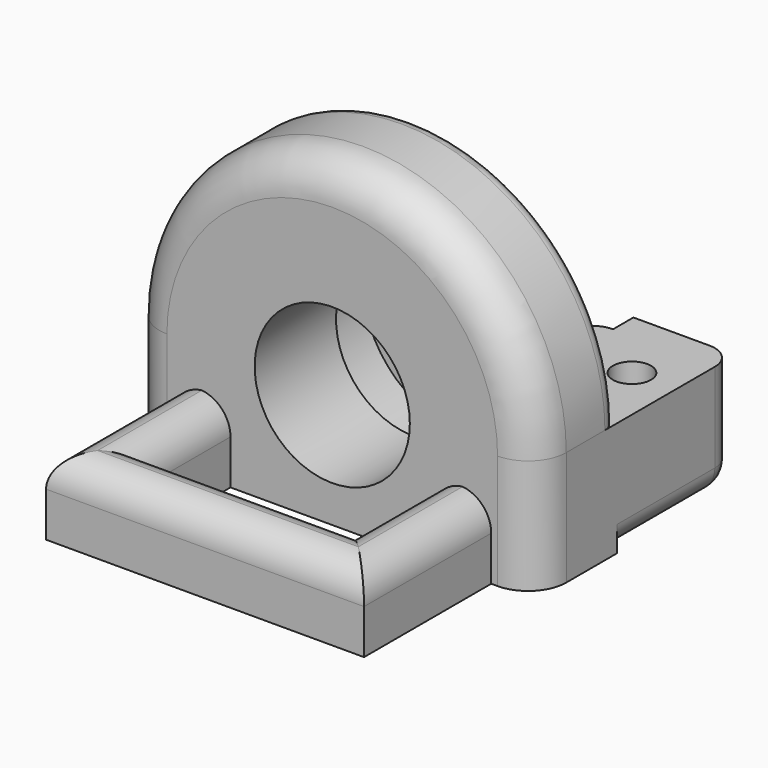
from build123d import *

# Parameters (mm, degrees)
F0_W          = 32
F0_H          = 11.6
F0_R          = 1.5
F1_DEPTH      = 9
F2_R          = 8
F1_FACE1_W    = 32
F1_FACE1_H    = 9
F3_DEPTH      = 5
F4_R          = 8
F5_DEPTH      = 2
F6_R          = 6
F7_DEPTH      = 25
F8_T1_DEPTH   = 28
F8_T3_DEPTH   = 12
F8_T5_DEPTH   = 14.6
F8_S9_W       = 2
F8_S9_H       = 2
F8_T10_DEPTH  = 2
F8_S15_W      = 2
F8_S15_H      = 2
F8_T16_DEPTH  = 2
F8_T20_ANGLE  = 275.6465366004
F10_DEPTH     = 8
F12_DEPTH     = 6
F13_T1_DEPTH  = 8
F13_T3_DEPTH  = 18.75
F13_T5_DEPTH  = 16
F13_T7_DEPTH  = 37.5
F13_T13_DEPTH = 14.25
F13_T17_DEPTH = 22.25
F13_T24_DEPTH = 14.25
F13_T28_DEPTH = 22.25
F14_R         = 3
F15_R         = 1.2
F16_R         = 6.1
F17_DEPTH     = 19.6010001
F18_T3_ANGLE  = 90
F18_T6_DEPTH  = 10
F18_T9_DEPTH  = 0.5


# Not quite as in the source:
# - a fillet or chamfer that OpenCascade refuses, or shapes differently, is made with other operations: its cross-section is extruded or revolved along the edge and cut away or added


with BuildPart() as f1:
    # F0 (on Top) → F1 (new body)
    with BuildSketch(Plane.XY):
        Rectangle(F0_W, F0_H)
        with Locations((-12.524, 0)):
            Circle(F0_R, mode=Mode.SUBTRACT)
        with Locations((12.524, 0)):
            Circle(F0_R, mode=Mode.SUBTRACT)
    extrude(amount=F1_DEPTH)

    # F2 (on face) + F1_face1 (on face) → F3 (cut)
    with BuildSketch(Plane.XZ.offset(5.8)):
        with Locations((0, 9)):
            Circle(F2_R)
    with BuildSketch(Plane(origin=(0, 5.8, 4.5), x_dir=(-1, 0, 0), z_dir=(0, 1, 0))):
        Rectangle(F1_FACE1_W, F1_FACE1_H)
    extrude(amount=-F3_DEPTH, dir=(0, -1, 0), mode=Mode.SUBTRACT)

    # F4 (on face) → F5 (cut)
    with BuildSketch(Plane(origin=(0, 5.8, 0), x_dir=(-1, 0, 0), z_dir=(0, 1, 0))):
        with Locations((0, 9)):
            Circle(F4_R)
    extrude(amount=-F5_DEPTH, mode=Mode.SUBTRACT)

    # F6 (on face) → F7 (cut)
    with BuildSketch(Plane(origin=(0, 3.8, 0), x_dir=(-1, 0, 0), z_dir=(0, 1, 0))):
        with Locations((0, 9)):
            Circle(F6_R)
    extrude(amount=-F7_DEPTH, mode=Mode.SUBTRACT)

    # F8: fillet of radius 2 on 6 edges, made by hand

    # F8_s2 → F8_t1 (cut)
    with BuildSketch(Plane.YZ.offset(-14)):
        with BuildLine():
            ThreePointArc((5.8, 2), (5.2142135624, 0.5857864376), (3.8, 0))
            Line((3.8, 0), (5.8, 0))
            Line((5.8, 0), (5.8, 2))
        make_face()
    extrude(amount=F8_T1_DEPTH, mode=Mode.SUBTRACT)

    # F8_s4 → F8_t3 (cut)
    with BuildSketch(Plane.XY.offset(2)):
        with BuildLine():
            ThreePointArc((-14, 5.8), (-15.4142135624, 5.2142135624), (-16, 3.8))
            Line((-16, 3.8), (-16, 5.8))
            Line((-16, 5.8), (-14, 5.8))
        make_face()
        with BuildLine():
            ThreePointArc((14, 5.8), (15.4142135624, 5.2142135624), (16, 3.8))
            Line((16, 3.8), (16, 5.8))
            Line((16, 5.8), (14, 5.8))
        make_face()
    extrude(amount=F8_T3_DEPTH, mode=Mode.SUBTRACT)

    # F8_s6 → F8_t5 (cut)
    with BuildSketch(Plane.XZ.offset(-3.8)):
        with BuildLine():
            ThreePointArc((-14, 0), (-15.4142135624, 0.5857864376), (-16, 2))
            Line((-16, 2), (-16, 0))
            Line((-16, 0), (-14, 0))
        make_face()
        with BuildLine():
            ThreePointArc((14, 0), (15.4142135624, 0.5857864376), (16, 2))
            Line((16, 2), (16, 0))
            Line((16, 0), (14, 0))
        make_face()
    extrude(amount=F8_T5_DEPTH, mode=Mode.SUBTRACT)


with BuildPart() as f8_tool8:
    # F8_s9 → F8_t10 (new body)
    with BuildSketch(Plane.XZ.offset(-3.8)):
        with Locations((15, 1)):
            Rectangle(F8_S9_W, F8_S9_H)
    extrude(amount=-F8_T10_DEPTH)

    # F8_s11 → F8_t12 (revolve, cut)
    with BuildSketch(Plane(origin=(14, 3.8, 2), x_dir=(-0.7071067812, 0, 0.7071067812), z_dir=(-0.7071067812, 0, -0.7071067812))):
        with BuildLine():
            ThreePointArc((0, -2), (2, 0), (0, 2))
            Line((0, 2), (0, -2))
        make_face()
    revolve(axis=Axis((14, 3.8, 2), (0, 1, 0)), mode=Mode.SUBTRACT)


with BuildPart() as f1_1:
    add(f1.part)

    # F8_t7: cut F8_tool8
    add(f8_tool8.part, mode=Mode.SUBTRACT)


with BuildPart() as f8_tool14:
    # F8_s15 → F8_t16 (new body)
    with BuildSketch(Plane.XZ.offset(-3.8)):
        with Locations((-15, 1)):
            Rectangle(F8_S15_W, F8_S15_H)
    extrude(amount=-F8_T16_DEPTH)

    # F8_s17 → F8_t18 (revolve, cut)
    with BuildSketch(Plane(origin=(-14, 3.8, 2), x_dir=(0.7071067812, 0, 0.7071067812), z_dir=(-0.7071067812, 0, 0.7071067812))):
        with BuildLine():
            ThreePointArc((0, -2), (2, 0), (0, 2))
            Line((0, 2), (0, -2))
        make_face()
    revolve(axis=Axis((-14, 3.8, 2), (0, 1, 0)), mode=Mode.SUBTRACT)


with BuildPart() as f1_2:
    add(f1_1.part)

    # F8_t13: cut F8_tool14
    add(f8_tool14.part, mode=Mode.SUBTRACT)

    # F8_s19 → F8_t20 (revolve, cut)
    with BuildSketch(Plane(origin=(-4.4781651596, 0, 4.057239564), x_dir=(0, 1, 0), z_dir=(-0.7410773266, 0, 0.6714196869))):
        with BuildLine():
            ThreePointArc((3.8, -14.6696959394), (3.2142135624, -13.255482377), (1.8, -12.6696959394))
            Line((1.8, -12.6696959394), (3.8, -12.6696959394))
            Line((3.8, -12.6696959394), (3.8, -14.6696959394))
        make_face()
    revolve(axis=Axis((0, 3.8, 9), (0, 1, 0)), revolution_arc=F8_T20_ANGLE, mode=Mode.SUBTRACT)

    # F9 (on face) → F10 (join)
    with BuildSketch(Plane.XZ.offset(5.8)):
        with BuildLine():
            Line((16, 0), (16, 9))
            ThreePointArc((16, 9), (0, 25), (-16, 9))
            Line((-16, 9), (-16, 0))
            Line((-16, 0), (-13.2287565553, 0))
            Line((-13.2287565553, 0), (0, 0))
            Line((0, 0), (13.2287565553, 0))
            Line((13.2287565553, 0), (16, 0))
        make_face()
    extrude(amount=F10_DEPTH)

    # F11 (on Top) → F12 (join)
    with BuildSketch(Plane.XY):
        Polygon((-8, -21.8), (-8, -13.8), (-12.5, -13.8), (-12.5, -26.3), (12.5, -26.3), (12.5, -13.8), (8, -13.8), (8, -21.8), align=None)
    extrude(amount=F12_DEPTH)

    # F13: fillet of radius 2.5 on 6 edges, made by hand

    # F13_s2 → F13_t1 (cut)
    with BuildSketch(Plane.XZ.offset(13.8)):
        with BuildLine():
            ThreePointArc((-10.5, 6), (-8.732233047, 5.267766953), (-8, 3.5))
            Line((-8, 3.5), (-8, 6))
            Line((-8, 6), (-10.5, 6))
        make_face()
        with BuildLine():
            ThreePointArc((10.5, 6), (8.732233047, 5.267766953), (8, 3.5))
            Line((8, 3.5), (8, 6))
            Line((8, 6), (10.5, 6))
        make_face()
    extrude(amount=F13_T1_DEPTH, mode=Mode.SUBTRACT)

    # F13_s4 → F13_t3 (cut)
    with BuildSketch(Plane.XZ.offset(13.8)):
        with BuildLine():
            ThreePointArc((-10, 6), (-11.767766953, 5.267766953), (-12.5, 3.5))
            Line((-12.5, 3.5), (-12.5, 6))
            Line((-12.5, 6), (-10, 6))
        make_face()
        with BuildLine():
            ThreePointArc((12.5, 3.5), (11.767766953, 5.267766953), (10, 6))
            Line((10, 6), (12.5, 6))
            Line((12.5, 6), (12.5, 3.5))
        make_face()
    extrude(amount=F13_T3_DEPTH, mode=Mode.SUBTRACT)

    # F13_s6 → F13_t5 (cut)
    with BuildSketch(Plane.YZ.offset(-8)):
        with BuildLine():
            ThreePointArc((-24.3, 6), (-22.532233047, 5.267766953), (-21.8, 3.5))
            Line((-21.8, 3.5), (-21.8, 6))
            Line((-21.8, 6), (-24.3, 6))
        make_face()
    extrude(amount=F13_T5_DEPTH, mode=Mode.SUBTRACT)

    # F13_s8 → F13_t7 (cut)
    with BuildSketch(Plane.YZ.offset(-18.75)):
        with BuildLine():
            ThreePointArc((-23.8, 6), (-25.567766953, 5.267766953), (-26.3, 3.5))
            Line((-26.3, 3.5), (-26.3, 6))
            Line((-26.3, 6), (-23.8, 6))
        make_face()
    extrude(amount=F13_T7_DEPTH, mode=Mode.SUBTRACT)


with BuildPart() as f13_tool11:
    # F13_s12 → F13_t13 (new body)
    with BuildSketch(Plane.XZ.offset(28.05)):
        with BuildLine():
            ThreePointArc((-10.5, 6), (-8.732233047, 5.267766953), (-8, 3.5))
            Line((-8, 3.5), (-8, 6))
            Line((-8, 6), (-10.5, 6))
        make_face()
    extrude(amount=-F13_T13_DEPTH)

    split(bisect_by=Plane.XZ.offset(21.8), keep=Keep.TOP)


with BuildPart() as f13_tool15:
    # F13_s16 → F13_t17 (new body)
    with BuildSketch(Plane.YZ.offset(8)):
        with BuildLine():
            ThreePointArc((-24.3, 6), (-22.532233047, 5.267766953), (-21.8, 3.5))
            Line((-21.8, 3.5), (-21.8, 6))
            Line((-21.8, 6), (-24.3, 6))
        make_face()
    extrude(amount=-F13_T17_DEPTH)

    split(bisect_by=Plane.YZ.offset(-8), keep=Keep.BOTTOM)


with BuildPart() as f13_tool11_1:
    add(f13_tool11.part)

    # F13_t19: intersect F13_tool15
    add(f13_tool15.part, mode=Mode.INTERSECT)


with BuildPart() as f1_3:
    add(f1_2.part)

    # F13_t9: cut F13_tool11
    add(f13_tool11_1.part, mode=Mode.SUBTRACT)


with BuildPart() as f13_tool22:
    # F13_s23 → F13_t24 (new body)
    with BuildSketch(Plane.XZ.offset(13.8)):
        with BuildLine():
            ThreePointArc((10.5, 6), (8.732233047, 5.267766953), (8, 3.5))
            Line((8, 3.5), (8, 6))
            Line((8, 6), (10.5, 6))
        make_face()
    extrude(amount=F13_T24_DEPTH)

    split(bisect_by=Plane.XZ.offset(21.8), keep=Keep.TOP)


with BuildPart() as f13_tool26:
    # F13_s27 → F13_t28 (new body)
    with BuildSketch(Plane.YZ.offset(14.25)):
        with BuildLine():
            ThreePointArc((-24.3, 6), (-22.532233047, 5.267766953), (-21.8, 3.5))
            Line((-21.8, 3.5), (-21.8, 6))
            Line((-21.8, 6), (-24.3, 6))
        make_face()
    extrude(amount=-F13_T28_DEPTH)

    split(bisect_by=Plane.YZ.offset(8), keep=Keep.TOP)


with BuildPart() as f13_tool22_1:
    add(f13_tool22.part)

    # F13_t30: intersect F13_tool26
    add(f13_tool26.part, mode=Mode.INTERSECT)


with BuildPart() as f1_4:
    add(f1_3.part)

    # F13_t20: cut F13_tool22
    add(f13_tool22_1.part, mode=Mode.SUBTRACT)

    # F14
    f14_edges = [f1_4.edges().sort_by_distance(p)[0] for p in [
        (0, -13.8, 25),
        (16, -13.8, 4.5),
    ]]
    fillet(f14_edges, radius=F14_R)

    # F15
    f15_edges = [f1_4.edges().sort_by_distance(p)[0] for p in [
        (0, -5.8, 25),
    ]]
    fillet(f15_edges, radius=F15_R)

    # F16 (on face) → F17 (cut, through all)
    with BuildSketch(Plane.XZ.offset(13.8)):
        with Locations((0, 9)):
            Circle(F16_R)
    extrude(amount=-F17_DEPTH, mode=Mode.SUBTRACT)

    # F18: fillet of radius 2 on 3 edges, made by hand


with BuildPart() as f18_tool1:
    # F18_s2 → F18_t3 (revolve)
    with BuildSketch(Plane.XZ.offset(10.8)):
        with BuildLine():
            ThreePointArc((-16, 2), (-15.4142135624, 0.5857864376), (-14, 0))
            Line((-14, 0), (-16, 0))
            Line((-16, 0), (-16, 2))
        make_face()
    revolve(axis=Axis((-13, -10.8, 0), (0, 0, 1)), revolution_arc=F18_T3_ANGLE)


with BuildPart() as f18_tool4:
    # F18_s5 → F18_t6 (new body)
    with BuildSketch(Plane.XZ.offset(0.8)):
        with BuildLine():
            ThreePointArc((-16, 2), (-15.4142135624, 0.5857864376), (-14, 0))
            Line((-14, 0), (-16, 0))
            Line((-16, 0), (-16, 2))
        make_face()
    extrude(amount=F18_T6_DEPTH)


with BuildPart() as f18_tool7:
    # F18_s8 → F18_t9 (new body)
    with BuildSketch(Plane.YZ.offset(-12.5)):
        with BuildLine():
            ThreePointArc((-13.8, 2), (-13.2142135624, 0.5857864376), (-11.8, 0))
            Line((-11.8, 0), (-13.8, 0))
            Line((-13.8, 0), (-13.8, 2))
        make_face()
    extrude(amount=-F18_T9_DEPTH)


with BuildPart() as f1_5:
    add(f1_4.part)

    # F18_t10: cut F18_tool1, F18_tool4, F18_tool7
    add([f18_tool1.part, f18_tool4.part, f18_tool7.part], mode=Mode.SUBTRACT)


solid = f1_5.part
